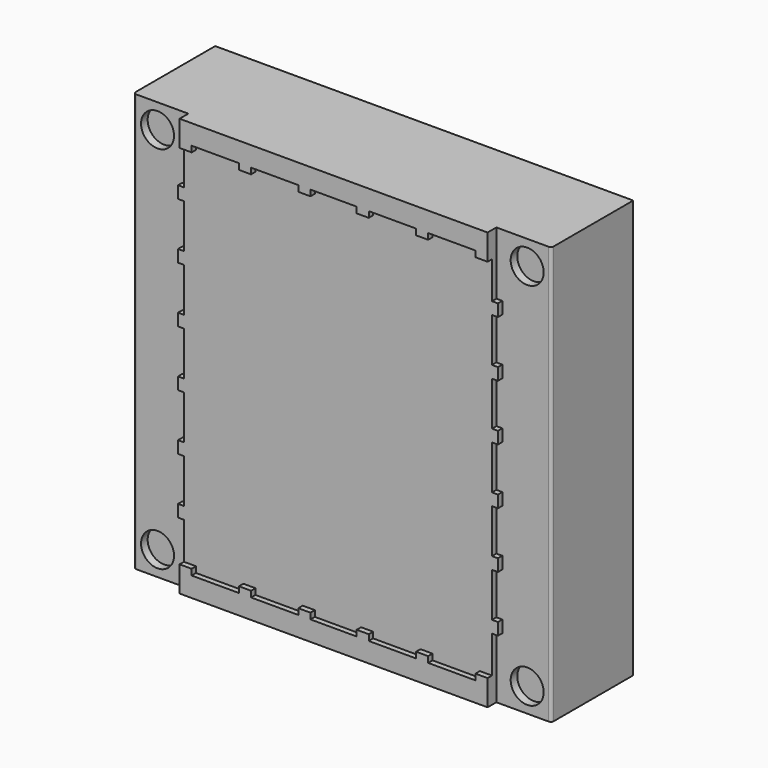
from build123d import *

# Parameters (mm, degrees)
F0_W      = 38
F0_H      = 38
F1_DEPTH  = 9.3
F2_R      = 1.5
F3_DEPTH  = 0.75
F5_DEPTH  = 0.5
F6_W      = 1.1
F6_H      = 0.54
F7_DEPTH  = 0.5
F8_R      = 0.25
F9_W      = 28
F9_H      = 28
F10_DEPTH = 5
F11_SIZE  = 0.5


with BuildPart() as f1:
    # F0 (on Front) → F1 (new body)
    with BuildSketch(Plane.XZ):
        Rectangle(F0_W, F0_H)
    extrude(amount=F1_DEPTH)

    # F2 (on face) → F3 (cut)
    with BuildSketch(Plane.XZ.offset(9.3)):
        with Locations((-16.8, 16.8)):
            Circle(F2_R)
        with Locations((16.8, 16.8)):
            Circle(F2_R)
        with Locations((16.8, -16.8)):
            Circle(F2_R)
        with Locations((-16.8, -16.8)):
            Circle(F2_R)
    extrude(amount=-F3_DEPTH, mode=Mode.SUBTRACT)

    # F4 (on face) → F5 (join)
    with BuildSketch(Plane.XZ.offset(9.3)):
        Polygon((14, 19), (0, 19), (-14, 19), (-14, 13.3), (-14.54, 13.3), (-14.54, 12.2), (-14, 12.2), (-14, 8.2), (-14.54, 8.2), (-14.54, 7.1), (-14, 7.1), (-14, 3.1), (-14.54, 3.1), (-14.54, 2), (-14, 2), (-14, -2), (-14.54, -2), (-14.54, -3.1), (-14, -3.1), (-14, -7.1), (-14.54, -7.1), (-14.54, -8.2), (-14, -8.2), (-14, -12.2), (-14.54, -12.2), (-14.54, -13.3), (-14, -13.3), (-14, -19), (0, -19), (14, -19), (14, -13.3), (14.54, -13.3), (14.54, -12.2), (14, -12.2), (14, -8.2), (14.54, -8.2), (14.54, -7.1), (14, -7.1), (14, -3.1), (14.54, -3.1), (14.54, -2), (14, -2), (14, 2), (14.54, 2), (14.54, 3.1), (14, 3.1), (14, 7.1), (14.54, 7.1), (14.54, 8.2), (14, 8.2), (14, 12.2), (14.54, 12.2), (14.54, 13.3), (14, 13.3), align=None)
    extrude(amount=F5_DEPTH)

    # F6 (on face) → F7 (join)
    with BuildSketch(Plane.XZ.offset(9.8)):
        Polygon((14, 17.2), (14, 19), (-14, 19), (-14, 17.2), (-12.9, 17.2), (-8.6, 17.2), (-7.5, 17.2), (-3.2, 17.2), (-2.1, 17.2), (2.1, 17.2), (3.2, 17.2), (7.5, 17.2), (8.6, 17.2), (12.9, 17.2), align=None)
        with Locations((13.45, 16.93)):
            Rectangle(F6_W, F6_H)
        with Locations((-13.45, 16.93)):
            Rectangle(F6_W, F6_H)
        with Locations((8.05, 16.93)):
            Rectangle(F6_W, F6_H)
        with Locations((-8.05, 16.93)):
            Rectangle(F6_W, F6_H)
        with Locations((2.65, 16.93)):
            Rectangle(F6_W, F6_H)
        with Locations((-2.65, 16.93)):
            Rectangle(F6_W, F6_H)
        with Locations((-13.45, -16.93)):
            Rectangle(F6_W, F6_H)
        Polygon((-12.9, -17.2), (-14, -17.2), (-14, -19), (14, -19), (14, -17.2), (12.9, -17.2), (8.6, -17.2), (7.5, -17.2), (3.2, -17.2), (2.1, -17.2), (-2.1, -17.2), (-3.2, -17.2), (-7.5, -17.2), (-8.6, -17.2), align=None)
        with Locations((-8.05, -16.93)):
            Rectangle(F6_W, F6_H)
        with Locations((13.45, -16.93)):
            Rectangle(F6_W, F6_H)
        with Locations((-2.65, -16.93)):
            Rectangle(F6_W, F6_H)
        with Locations((8.05, -16.93)):
            Rectangle(F6_W, F6_H)
        with Locations((2.65, -16.93)):
            Rectangle(F6_W, F6_H)
    extrude(amount=F7_DEPTH)

    # F8
    f8_edges = [f1.edges().sort_by_distance(p)[0] for p in [
        (-19, -9.3, 0),
        (19, -9.3, 0),
    ]]
    fillet(f8_edges, radius=F8_R)

    # F9 (on face) → F10 (cut)
    with BuildSketch(Plane.XZ):
        Rectangle(F9_W, F9_H)
    extrude(amount=F10_DEPTH, mode=Mode.SUBTRACT)

    # F11
    f11_edges = [f1.edges().sort_by_distance(p)[0] for p in [
        (-14, -2.5, 14),
        (0, -5, 14),
        (-14, -5, 0),
        (14, -2.5, 14),
        (14, -2.5, -14),
        (14, 0, 0),
        (14, -5, 0),
        (-14, -2.5, -14),
        (0, 0, -14),
        (0, -5, -14),
        (0, 0, 14),
        (-14, 0, 0),
    ]]
    chamfer(f11_edges, length=F11_SIZE)


solid = f1.part
